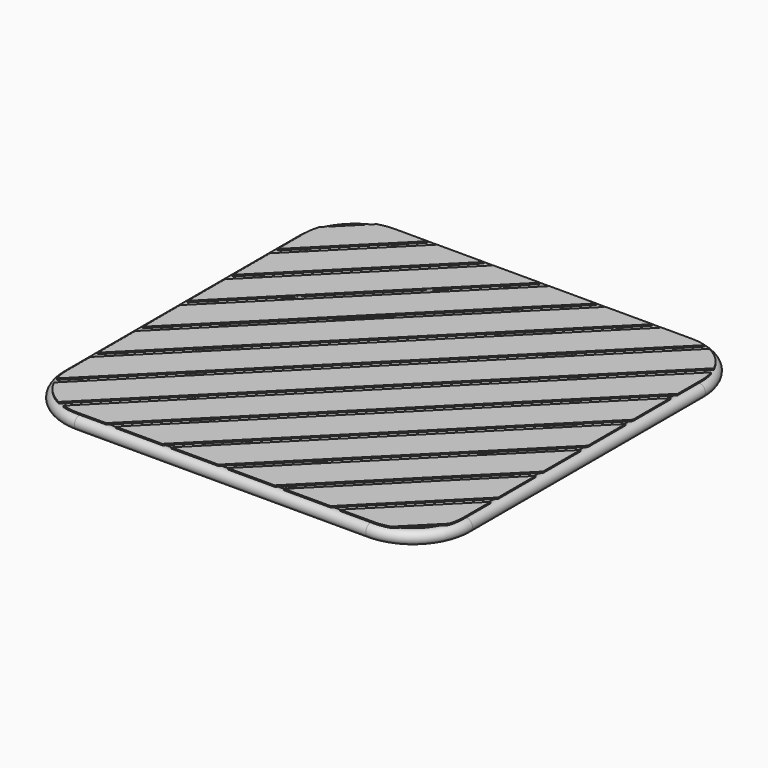
from build123d import *

# Parameters (mm, degrees)
F1_R          = 9.5
F1_R_2        = 7.5
F5_DEPTH      = 2
F5_DEPTH_BACK = 0.1
F6_R          = 232
F6_R_2        = 229
F7_DEPTH      = 40


# Not quite as in the source:
# - a feature names something its author has since deleted; it is built from what else it names


with BuildPart() as f2:
    # F2: sweep along a path in F0
    with BuildLine(Plane.XY) as f2_path:
        Line((-300, 220), (-300, -220))
        ThreePointArc((-300, -220), (-276.5685424949, -276.5685424949), (-220, -300))
        Line((-220, -300), (220, -300))
        ThreePointArc((220, -300), (276.5685424949, -276.5685424949), (300, -220))
        Line((300, -220), (300, 220))
        ThreePointArc((300, 220), (276.5685424949, 276.5685424949), (220, 300))
        Line((220, 300), (-220, 300))
        ThreePointArc((-220, 300), (-276.5685424949, 276.5685424949), (-300, 220))
    # F1 (on Front) → F2 (sweep)
    with BuildSketch(Plane.XZ):
        with Locations((-299.9776005745, 0)):
            Circle(F1_R)
        with Locations((-299.9776005745, 0)):
            Circle(F1_R_2, mode=Mode.SUBTRACT)
    sweep(path=f2_path.line)

    # F4 (on offset) → F5 (join, two sides)
    with BuildSketch(Plane.XY.offset(9.5)) as f5_sk:
        Polygon((-4.0559159102, 300), (-74.7665940289, 300), (-300, 74.7665940289), (-300, 4.0559159102), align=None)
        Polygon((80.7968978322, 300), (10.0862197135, 300), (-300, -10.0862197135), (-300, -80.7968978322), align=None)
        Polygon((165.6497115746, 300), (94.9390334559, 300), (-300, -94.9390334559), (-300, -165.6497115746), align=None)
        with BuildLine():
            Line((225, 300), (179.7918471983, 300))
            Line((179.7918471983, 300), (-300, -179.7918471983))
            Line((-300, -179.7918471983), (-300, -225))
            ThreePointArc((-300, -225), (-299.1585029531, -236.2034119695), (-296.6528949398, -247.1554202567))
            Line((-296.6528949398, -247.1554202567), (247.1554202567, 296.6528949398))
            ThreePointArc((247.1554202567, 296.6528949398), (236.2034119695, 299.1585029531), (225, 300))
        make_face()
        with BuildLine():
            ThreePointArc((300, 225), (299.1585029531, 236.2034119695), (296.6528949398, 247.1554202567))
            Line((296.6528949398, 247.1554202567), (-247.1554202567, -296.6528949398))
            ThreePointArc((-247.1554202567, -296.6528949398), (-236.2034119695, -299.1585029531), (-225, -300))
            Line((-225, -300), (-179.7918471983, -300))
            Line((-179.7918471983, -300), (300, 179.7918471983))
            Line((300, 179.7918471983), (300, 225))
        make_face()
        Polygon((300, 94.9390334559), (300, 165.6497115746), (-165.6497115746, -300), (-94.9390334559, -300), align=None)
        Polygon((300, 10.0862197135), (300, 80.7968978322), (-80.7968978322, -300), (-10.0862197135, -300), align=None)
        Polygon((300, -74.7665940289), (300, -4.0559159102), (4.0559159102, -300), (74.7665940289, -300), align=None)
        Polygon((300, -159.6194077713), (300, -88.9087296526), (88.9087296526, -300), (159.6194077713, -300), align=None)
        with BuildLine():
            Line((300, -225), (300, -173.761543395))
            Line((300, -173.761543395), (173.761543395, -300))
            Line((173.761543395, -300), (225, -300))
            ThreePointArc((225, -300), (236.7069941389, -299.0806741886), (248.1269871608, -296.3452343529))
            Line((248.1269871608, -296.3452343529), (296.3452343529, -248.1269871608))
            ThreePointArc((296.3452343529, -248.1269871608), (299.0806741886, -236.7069941389), (300, -225))
        make_face()
        Polygon((-88.9087296526, 300), (-159.6194077713, 300), (-300, 159.6194077713), (-300, 88.9087296526), align=None)
        with BuildLine():
            Line((-173.761543395, 300), (-225, 300))
            ThreePointArc((-225, 300), (-236.7069941389, 299.0806741886), (-248.1269871608, 296.3452343529))
            Line((-248.1269871608, 296.3452343529), (-296.3452343529, 248.1269871608))
            ThreePointArc((-296.3452343529, 248.1269871608), (-299.0806741886, 236.7069941389), (-300, 225))
            Line((-300, 225), (-300, 173.761543395))
            Line((-300, 173.761543395), (-173.761543395, 300))
        make_face()
        with BuildLine():
            ThreePointArc((292.6776695297, 257.3223304703), (278.033008589, 278.033008589), (257.3223304703, 292.6776695297))
            Line((257.3223304703, 292.6776695297), (-292.6776695297, -257.3223304703))
            ThreePointArc((-292.6776695297, -257.3223304703), (-278.033008589, -278.033008589), (-257.3223304703, -292.6776695297))
            Line((-257.3223304703, -292.6776695297), (292.6776695297, 257.3223304703))
        make_face()
    extrude(amount=F5_DEPTH)
    extrude(f5_sk.sketch, amount=-F5_DEPTH_BACK)

    # F6 (on face) → F7 (join)
    with BuildSketch(Plane(origin=(0, 0, 9.4), x_dir=(1, 0, 0), z_dir=(0, 0, -1))):
        Circle(F6_R)
        Circle(F6_R_2, mode=Mode.SUBTRACT)
    extrude(amount=F7_DEPTH)


solid = f2.part
